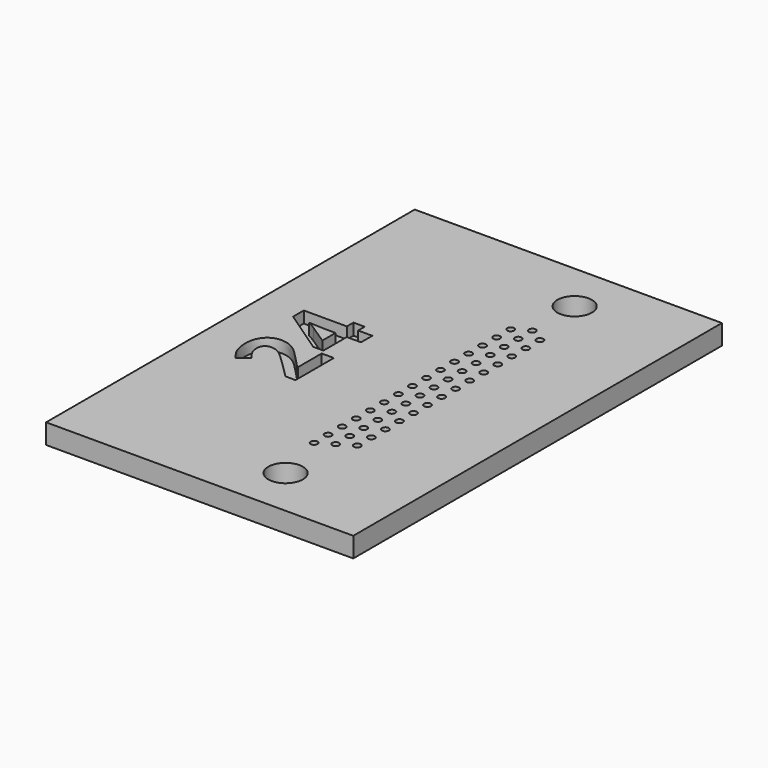
from build123d import *

# Parameters (mm, degrees)
F0_W         = 40
F0_H         = 60
F1_DEPTH     = 2.6
F2_TEXT_SIZE = 12.5
F3_DEPTH     = 1.5
F4_R         = 0.45
F4_R_2       = 2.25
F5_DEPTH     = 2.6


# Not quite as in the source:
# - Text() gives the source's letters only with a copy of the font that has no kerning and outlines rounded to 1/6400 em; it was checked with that copy


with BuildPart() as f1:
    # F0 (on Top) → F1 (new body)
    with BuildSketch(Plane.XY):
        with Locations((-23.1587231159, 8.3350909071)):
            Rectangle(F0_W, F0_H)
    extrude(amount=F1_DEPTH)

    # F2 (on face) → F3 (cut)
    with BuildSketch(Plane.XY.offset(2.6)):
        with Locations(Location((-29.1587231159, 0.9350909071), (0, 0, 90))):
            Text('24', F2_TEXT_SIZE, font='Open Sans', font_style=FontStyle.BOLD, text_align=(TextAlign.LEFT, TextAlign.BOTTOM))
    extrude(amount=-F3_DEPTH, mode=Mode.SUBTRACT)

    # F4 (on face) → F5 (cut, through all)
    with BuildSketch(Plane.XY.offset(2.6)):
        with Locations((-19.0587231159, 14.6900909071)):
            Circle(F4_R)
        with Locations((-19.0587231159, 16.9760909071)):
            Circle(F4_R)
        with Locations((-19.0587231159, 19.2620909071)):
            Circle(F4_R)
        with Locations((-19.0587231159, 21.5480909071)):
            Circle(F4_R)
        with Locations((-19.0587231159, 23.8340909071)):
            Circle(F4_R)
        with Locations((-17.1587231159, 15.8330909071)):
            Circle(F4_R)
        with Locations((-17.1587231159, 18.1190909071)):
            Circle(F4_R)
        with Locations((-17.1587231159, 20.4050909071)):
            Circle(F4_R)
        with Locations((-17.1587231159, 22.6910909071)):
            Circle(F4_R)
        with Locations((-17.1587231159, 24.9770909071)):
            Circle(F4_R)
        with Locations((-15.2587231159, 14.6900909071)):
            Circle(F4_R)
        with Locations((-15.2587231159, 16.9760909071)):
            Circle(F4_R)
        with Locations((-15.2587231159, 19.2620909071)):
            Circle(F4_R)
        with Locations((-15.2587231159, 21.5480909071)):
            Circle(F4_R)
        with Locations((-15.2587231159, 23.8340909071)):
            Circle(F4_R)
        with Locations((-19.0587231159, 3.2600909071)):
            Circle(F4_R)
        with Locations((-19.0587231159, 5.5460909071)):
            Circle(F4_R)
        with Locations((-19.0587231159, 7.8320909071)):
            Circle(F4_R)
        with Locations((-19.0587231159, 10.1180909071)):
            Circle(F4_R)
        with Locations((-19.0587231159, 12.4040909071)):
            Circle(F4_R)
        with Locations((-17.1587231159, 4.4030909071)):
            Circle(F4_R)
        with Locations((-17.1587231159, 6.6890909071)):
            Circle(F4_R)
        with Locations((-17.1587231159, 8.9750909071)):
            Circle(F4_R)
        with Locations((-17.1587231159, 11.2610909071)):
            Circle(F4_R)
        with Locations((-17.1587231159, 13.5470909071)):
            Circle(F4_R)
        with Locations((-15.2587231159, 3.2600909071)):
            Circle(F4_R)
        with Locations((-15.2587231159, 5.5460909071)):
            Circle(F4_R)
        with Locations((-15.2587231159, 7.8320909071)):
            Circle(F4_R)
        with Locations((-15.2587231159, 10.1180909071)):
            Circle(F4_R)
        with Locations((-15.2587231159, 12.4040909071)):
            Circle(F4_R)
        with Locations((-19.0587231159, -8.1699090929)):
            Circle(F4_R)
        with Locations((-19.0587231159, -5.8839090929)):
            Circle(F4_R)
        with Locations((-19.0587231159, -3.5979090929)):
            Circle(F4_R)
        with Locations((-19.0587231159, -1.3119090929)):
            Circle(F4_R)
        with Locations((-19.0587231159, 0.9740909071)):
            Circle(F4_R)
        with Locations((-17.1587231159, -7.0269090929)):
            Circle(F4_R)
        with Locations((-17.1587231159, -4.7409090929)):
            Circle(F4_R)
        with Locations((-17.1587231159, -2.4549090929)):
            Circle(F4_R)
        with Locations((-17.1587231159, -0.1689090929)):
            Circle(F4_R)
        with Locations((-17.1587231159, 2.1170909071)):
            Circle(F4_R)
        with Locations((-15.2587231159, -5.8839090929)):
            Circle(F4_R)
        with Locations((-15.2587231159, -3.5979090929)):
            Circle(F4_R)
        with Locations((-15.2587231159, -1.3119090929)):
            Circle(F4_R)
        with Locations((-15.2587231159, 0.9740909071)):
            Circle(F4_R)
        with Locations((-17.1587231159, 31.8600909071)):
            Circle(F4_R_2)
        with Locations((-17.1587231159, -15.1799090929)):
            Circle(F4_R_2)
    extrude(amount=-F5_DEPTH, mode=Mode.SUBTRACT)


solid = f1.part
